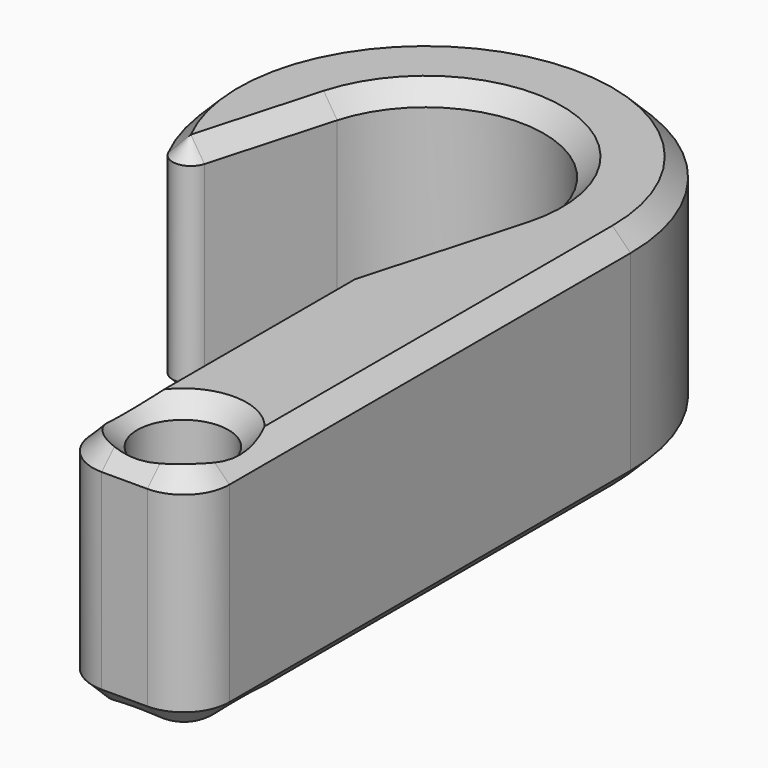
from build123d import *

# Parameters (mm, degrees)
F0_R         = 5
F1_DEPTH     = 25
F2_R         = 5
F3_R         = 2
F4_T1_DEPTH  = 13.9731886125
F4_T3_DEPTH  = 27.1080898313
F4_T5_DEPTH  = 55
F4_T7_DEPTH  = 42.5305187235
F4_T9_DEPTH  = 5
F4_T12_ANGLE = 137.0297160683
F4_T14_ANGLE = 180
F4_T16_ANGLE = 207.1471098896
F4_T18_ANGLE = 90
F4_T20_ANGLE = 90
F4_T24_ANGLE = 137.0297160683
F4_T26_ANGLE = 180
F4_T28_ANGLE = 207.1471098896
F4_T30_ANGLE = 90
F4_T32_ANGLE = 90


# Not quite as in the source:
# - a fillet or chamfer that OpenCascade refuses, or shapes differently, is made with other operations: its cross-section is extruded or revolved along the edge and cut away or added


with BuildPart() as f1:
    # F0 (on Top) → F1 (new body)
    with BuildSketch(Plane.XY):
        with BuildLine():
            ThreePointArc((7.5, -21.2132034356), (18.3711730709, -12.9903810568), (22.5, 0))
            ThreePointArc((22.5, 0), (-7.4888899158, 21.2171281711), (-17.5148024737, -14.1237988625))
            Line((-17.5148024737, -14.1237988625), (-12.5074012369, 3.5447022866))
            ThreePointArc((-12.5074012369, 3.5447022866), (1.7893831229, 12.8762614155), (13, 0))
            ThreePointArc((13, 0), (12.8762614155, -1.7893831229), (12.5074012369, -3.5447022866))
            Line((12.5074012369, -3.5447022866), (7.5, -21.2132034356))
        make_face()
        with BuildLine():
            Line((22.5, -60), (22.5, 0))
            ThreePointArc((22.5, 0), (18.3711730709, -12.9903810568), (7.5, -21.2132034356))
            Line((7.5, -21.2132034356), (7.5, -60))
            Line((7.5, -60), (22.5, -60))
        make_face()
        with Locations((15, -52)):
            Circle(F0_R, mode=Mode.SUBTRACT)
    extrude(amount=F1_DEPTH)

    # F2
    f2_edges = [f1.edges().sort_by_distance(p)[0] for p in [
        (22.5, -60, 12.5),
        (7.5, -60, 12.5),
    ]]
    fillet(f2_edges, radius=F2_R)

    # F3
    f3_edges = [f1.edges().sort_by_distance(p)[0] for p in [
        (-17.514802, -14.123799, 12.5),
    ]]
    fillet(f3_edges, radius=F3_R)

    # F4: chamfer of 2 on 22 edges, made by hand

    # F4_s2 → F4_t1 (cut)
    with BuildSketch(Plane(origin=(-3.8100610481, -13.4437135796, 0), x_dir=(0, 0, 1), z_dir=(0.2726694067, 0.9621077875, 0))):
        Polygon((23, -13), (25, -15), (25, -13), align=None)
        Polygon((0, -15), (2, -13), (0, -13), align=None)
    extrude(amount=F4_T1_DEPTH, mode=Mode.SUBTRACT)

    # F4_s4 → F4_t3 (cut)
    with BuildSketch(Plane(origin=(0, 0, 0), x_dir=(0, 0, 1), z_dir=(-0.2726694067, -0.9621077875, 0))):
        Polygon((23, -13), (25, -15), (25, -13), align=None)
        Polygon((0, -15), (2, -13), (0, -13), align=None)
    extrude(amount=F4_T3_DEPTH, mode=Mode.SUBTRACT)

    # F4_s6 → F4_t5 (cut)
    with BuildSketch(Plane.XZ):
        Polygon((22.5, 23), (20.5, 25), (22.5, 25), align=None)
        Polygon((20.5, 0), (22.5, 2), (22.5, 0), align=None)
    extrude(amount=F4_T5_DEPTH, mode=Mode.SUBTRACT)

    # F4_s8 → F4_t7 (cut)
    with BuildSketch(Plane.XZ.offset(12.4694812765)):
        Polygon((7.5, 23), (9.5, 25), (7.5, 25), align=None)
        Polygon((9.5, 0), (7.5, 2), (7.5, 0), align=None)
    extrude(amount=F4_T7_DEPTH, mode=Mode.SUBTRACT)

    # F4_s10 → F4_t9 (cut)
    with BuildSketch(Plane.YZ.offset(12.5)):
        Polygon((-60, 23), (-58, 25), (-60, 25), align=None)
        Polygon((-58, 0), (-60, 2), (-60, 0), align=None)
    extrude(amount=F4_T9_DEPTH, mode=Mode.SUBTRACT)

    # F4_s11 → F4_t12 (revolve, cut)
    with BuildSketch(Plane(origin=(-3.8100610481, -13.4437135796, 0), x_dir=(0, 0, 1), z_dir=(0.2726694067, 0.9621077875, 0))):
        Polygon((23, -13), (25, -15), (25, -13), align=None)
    revolve(axis=Axis((-18.2416778599, -9.3536724797, 25), (0, 0, -1)), revolution_arc=F4_T12_ANGLE, mode=Mode.SUBTRACT)

    # F4_s13 → F4_t14 (revolve, cut)
    with BuildSketch(Plane(origin=(0, 0, 0), x_dir=(0, 0, 1), z_dir=(-0.2726694067, -0.9621077875, 0))):
        Polygon((23, 13), (25, 15), (25, 13), align=None)
    revolve(axis=Axis((0, 0, 25), (0, 0, -1)), revolution_arc=F4_T14_ANGLE, mode=Mode.SUBTRACT)

    # F4_s15 → F4_t16 (revolve, cut)
    with BuildSketch(Plane.XZ):
        Polygon((22.5, 23), (20.5, 25), (22.5, 25), align=None)
    revolve(axis=Axis((0, 0, 25), (0, 0, 1)), revolution_arc=F4_T16_ANGLE, mode=Mode.SUBTRACT)

    # F4_s17 → F4_t18 (revolve, cut)
    with BuildSketch(Plane.YZ.offset(17.5)):
        Polygon((-60, 23), (-58, 25), (-60, 25), align=None)
    revolve(axis=Axis((17.5, -55, 25), (0, 0, 1)), revolution_arc=F4_T18_ANGLE, mode=Mode.SUBTRACT)

    # F4_s19 → F4_t20 (revolve, cut)
    with BuildSketch(Plane.XZ.offset(55)):
        Polygon((7.5, 23), (9.5, 25), (7.5, 25), align=None)
    revolve(axis=Axis((12.5, -55, 25), (0, 0, 1)), revolution_arc=F4_T20_ANGLE, mode=Mode.SUBTRACT)

    # F4_s21 → F4_t22 (revolve, cut)
    with BuildSketch(Plane.XZ.offset(52)):
        Polygon((20, 23), (22, 25), (20, 25), align=None)
    revolve(axis=Axis((15, -52, 25), (0, 0, 1)), mode=Mode.SUBTRACT)

    # F4_s23 → F4_t24 (revolve, cut)
    with BuildSketch(Plane(origin=(-3.8100610481, -13.4437135796, 0), x_dir=(0, 0, 1), z_dir=(0.2726694067, 0.9621077875, 0))):
        Polygon((0, -15), (2, -13), (0, -13), align=None)
    revolve(axis=Axis((-18.2416778599, -9.3536724797, 0), (0, 0, -1)), revolution_arc=F4_T24_ANGLE, mode=Mode.SUBTRACT)

    # F4_s25 → F4_t26 (revolve, cut)
    with BuildSketch(Plane(origin=(0, 0, 0), x_dir=(0, 0, 1), z_dir=(-0.2726694067, -0.9621077875, 0))):
        Polygon((0, 15), (2, 13), (0, 13), align=None)
    revolve(axis=Axis((0, 0, 0), (0, 0, -1)), revolution_arc=F4_T26_ANGLE, mode=Mode.SUBTRACT)

    # F4_s27 → F4_t28 (revolve, cut)
    with BuildSketch(Plane.XZ):
        Polygon((20.5, 0), (22.5, 2), (22.5, 0), align=None)
    revolve(axis=Axis((0, 0, 0), (0, 0, 1)), revolution_arc=F4_T28_ANGLE, mode=Mode.SUBTRACT)

    # F4_s29 → F4_t30 (revolve, cut)
    with BuildSketch(Plane.YZ.offset(17.5)):
        Polygon((-58, 0), (-60, 2), (-60, 0), align=None)
    revolve(axis=Axis((17.5, -55, 0), (0, 0, 1)), revolution_arc=F4_T30_ANGLE, mode=Mode.SUBTRACT)

    # F4_s31 → F4_t32 (revolve, cut)
    with BuildSketch(Plane.XZ.offset(55)):
        Polygon((9.5, 0), (7.5, 2), (7.5, 0), align=None)
    revolve(axis=Axis((12.5, -55, 0), (0, 0, 1)), revolution_arc=F4_T32_ANGLE, mode=Mode.SUBTRACT)

    # F4_s33 → F4_t34 (revolve, cut)
    with BuildSketch(Plane.XZ.offset(52)):
        Polygon((22, 0), (20, 2), (20, 0), align=None)
    revolve(axis=Axis((15, -52, 0), (0, 0, 1)), mode=Mode.SUBTRACT)


solid = f1.part
